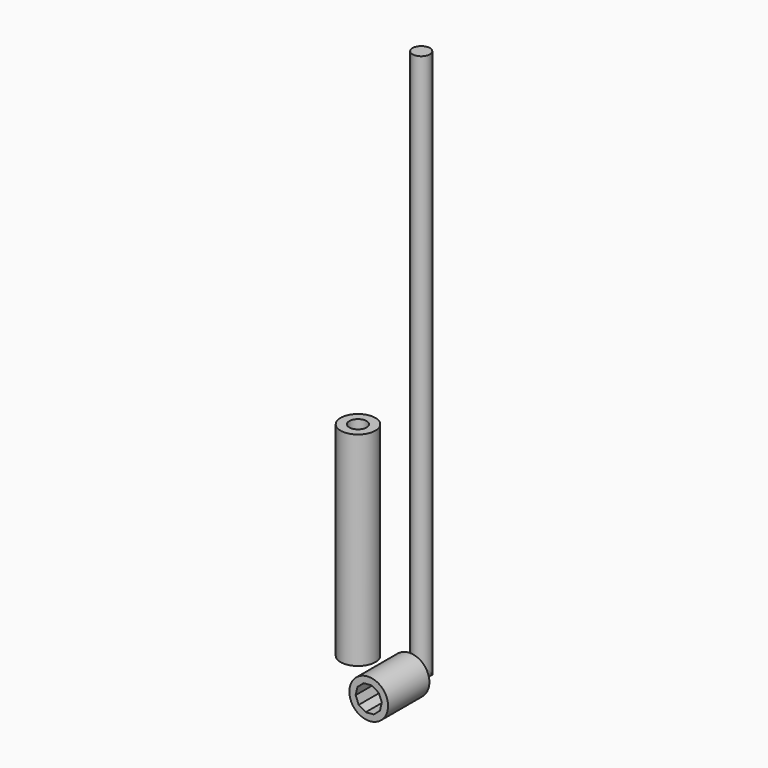
from build123d import *

# Parameters (mm, degrees)
F0_R      = 14.25
F1_DEPTH  = 38
F3_DEPTH  = 40
F4_DEPTH  = 12
F6_DEPTH  = 15
F7_R      = 6.35
F10_R     = 12.8
F10_R_2   = 6.4
F11_DEPTH = 150
F12_DEPTH = 12


with BuildPart() as f1:
    # F0 (on Front) → F1 (new body)
    with BuildSketch(Plane.XZ):
        Circle(F0_R)
    extrude(amount=F1_DEPTH)

    # F2 (on Front) → F3 (cut)
    with BuildSketch(Plane.XZ):
        Polygon((3.7324627706, -8.9243713627), (8.2652396853, -5.0260815253), (9.6409759653, 0.7920006246), (7.3341871114, 6.307565455), (2.2259880607, 9.4138546678), (-3.7324627706, 8.9243713627), (-8.2652396853, 5.0260815253), (-9.6409759653, -0.7920006246), (-7.3341871114, -6.307565455), (-2.2259880607, -9.4138546678), align=None)
    extrude(amount=F3_DEPTH, mode=Mode.SUBTRACT)

    # F2 (on Front) → F4 (join)
    with BuildSketch(Plane.XZ):
        Polygon((3.7324627706, -8.9243713627), (8.2652396853, -5.0260815253), (9.6409759653, 0.7920006246), (7.3341871114, 6.307565455), (2.2259880607, 9.4138546678), (-3.7324627706, 8.9243713627), (-8.2652396853, 5.0260815253), (-9.6409759653, -0.7920006246), (-7.3341871114, -6.307565455), (-2.2259880607, -9.4138546678), align=None)
    extrude(amount=F4_DEPTH)

    # F5 (on Front) → F6 (cut)
    with BuildSketch(Plane.XZ):
        Polygon((-0.588765686, -9.0317968847), (9.0317968847, -0.588765686), (0.588765686, 9.0317968847), (-9.0317968847, 0.588765686), align=None)
    extrude(amount=F6_DEPTH, mode=Mode.SUBTRACT)


with BuildPart() as f9:
    # F9: sweep along a path in F8
    with BuildLine(Plane.YZ) as f9_path:
        Line((10.325, 400), (10.325, 0))
        Line((10.325, 0), (0, 0))
    # F7 (on Front) → F9 (sweep)
    with BuildSketch(Plane.XZ):
        Circle(F7_R)
    sweep(path=f9_path.line, transition=Transition.RIGHT)

    # F7 (on Front) → F12 (join)
    with BuildSketch(Plane.XZ):
        Circle(F7_R)
    extrude(amount=F12_DEPTH)


with BuildPart() as f11:
    # F10 (on Top) → F11 (new body)
    with BuildSketch(Plane.XY):
        with Locations((-38.3003803454, 0)):
            Circle(F10_R)
        with Locations((-38.3003803454, 0)):
            Circle(F10_R_2, mode=Mode.SUBTRACT)
    extrude(amount=F11_DEPTH)


solid = Compound([f1.part, f9.part, f11.part])
